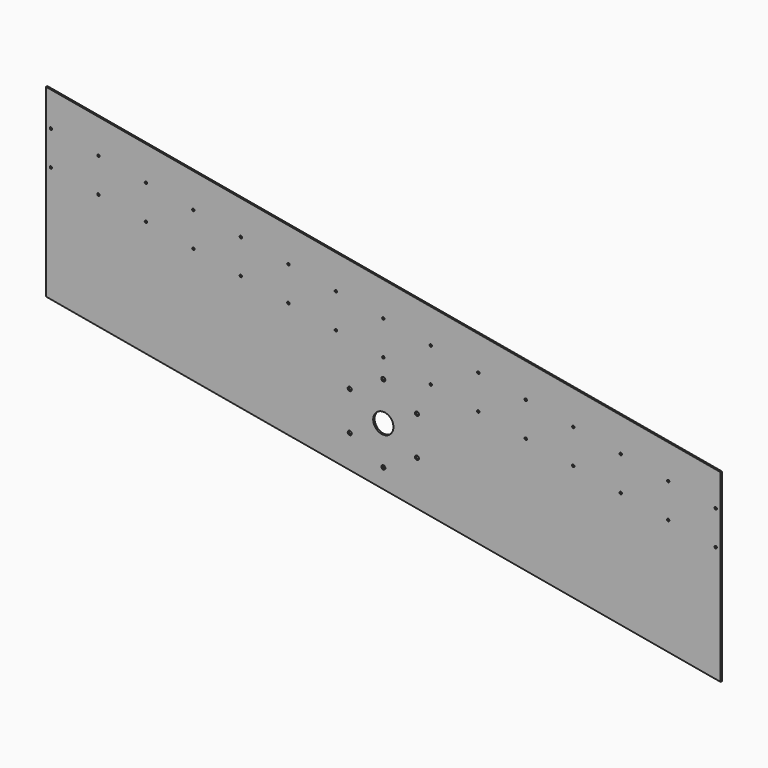
from build123d import *

# Parameters (mm, degrees)
F0_R     = 6
F0_R_2   = 30
F0_R_3   = 3.5
F1_DEPTH = 2.5


# Not quite as in the source:
# - a feature names something its author has since deleted; it is built from what else it names


with BuildPart() as f1:
    # F0 (on Front) → F1 (new body, symmetric)
    with BuildSketch(Plane.XZ):
        Polygon((0, 255), (1435, 0), (1435, 547.5993031359), (-565, 903), (-565, 355.4006968641), align=None)
        with Locations((335.4070785648, 292.4334004787)):
            Circle(F0_R, mode=Mode.SUBTRACT)
        with Locations((335.4070785648, 407.4334004787)):
            Circle(F0_R, mode=Mode.SUBTRACT)
        with Locations((435, 234.9334004787)):
            Circle(F0_R, mode=Mode.SUBTRACT)
        with Locations((534.5929214352, 292.4334004787)):
            Circle(F0_R, mode=Mode.SUBTRACT)
        with Locations((435, 349.9334004787)):
            Circle(F0_R_2, mode=Mode.SUBTRACT)
        with Locations((534.5929214352, 407.4334004787)):
            Circle(F0_R, mode=Mode.SUBTRACT)
        with Locations((857.3829507159, 447.1088550113)):
            Circle(F0_R_3, mode=Mode.SUBTRACT)
        with Locations((998.1772676211, 422.08965584)):
            Circle(F0_R_3, mode=Mode.SUBTRACT)
        with Locations((1138.9715845264, 397.0704566686)):
            Circle(F0_R_3, mode=Mode.SUBTRACT)
        with Locations((1279.7659014317, 372.0512574973)):
            Circle(F0_R_3, mode=Mode.SUBTRACT)
        with Locations((1420.560218337, 347.032058326)):
            Circle(F0_R_3, mode=Mode.SUBTRACT)
        with Locations((1420.560218337, 448.5986578473)):
            Circle(F0_R_3, mode=Mode.SUBTRACT)
        with Locations((-409.7659014317, 672.2816475532)):
            Circle(F0_R_3, mode=Mode.SUBTRACT)
        with Locations((-268.9715845264, 647.2624483819)):
            Circle(F0_R_3, mode=Mode.SUBTRACT)
        with Locations((-128.1772676211, 622.2432492105)):
            Circle(F0_R_3, mode=Mode.SUBTRACT)
        with Locations((294.2056830947, 547.1856516966)):
            Circle(F0_R_3, mode=Mode.SUBTRACT)
        with Locations((12.6170492841, 597.2240500392)):
            Circle(F0_R_3, mode=Mode.SUBTRACT)
        with Locations((153.4113661894, 572.2048508679)):
            Circle(F0_R_3, mode=Mode.SUBTRACT)
        with Locations((153.4113661894, 673.7714503892)):
            Circle(F0_R_3, mode=Mode.SUBTRACT)
        with Locations((294.2056830947, 648.7522512179)):
            Circle(F0_R_3, mode=Mode.SUBTRACT)
        with Locations((-550.560218337, 697.3008467245)):
            Circle(F0_R_3, mode=Mode.SUBTRACT)
        with Locations((-409.7659014317, 773.8482470745)):
            Circle(F0_R_3, mode=Mode.SUBTRACT)
        with Locations((-128.1772676211, 723.8098487319)):
            Circle(F0_R_3, mode=Mode.SUBTRACT)
        with Locations((-268.9715845264, 748.8290479032)):
            Circle(F0_R_3, mode=Mode.SUBTRACT)
        with Locations((-550.560218337, 798.8674462459)):
            Circle(F0_R_3, mode=Mode.SUBTRACT)
        with Locations((12.6170492841, 698.7906495606)):
            Circle(F0_R_3, mode=Mode.SUBTRACT)
        with Locations((435, 464.9334004787)):
            Circle(F0_R, mode=Mode.SUBTRACT)
        with Locations((575.7943169053, 497.1472533539)):
            Circle(F0_R_3, mode=Mode.SUBTRACT)
        with Locations((435, 522.1664525253)):
            Circle(F0_R_3, mode=Mode.SUBTRACT)
        with Locations((716.5886338106, 472.1280541826)):
            Circle(F0_R_3, mode=Mode.SUBTRACT)
        with Locations((857.3829507159, 548.6754545326)):
            Circle(F0_R_3, mode=Mode.SUBTRACT)
        with Locations((575.7943169053, 598.7138528753)):
            Circle(F0_R_3, mode=Mode.SUBTRACT)
        with Locations((435, 623.7330520466)):
            Circle(F0_R_3, mode=Mode.SUBTRACT)
        with Locations((716.5886338106, 573.694653704)):
            Circle(F0_R_3, mode=Mode.SUBTRACT)
        with Locations((1138.9715845264, 498.63705619)):
            Circle(F0_R_3, mode=Mode.SUBTRACT)
        with Locations((998.1772676211, 523.6562553613)):
            Circle(F0_R_3, mode=Mode.SUBTRACT)
        with Locations((1279.7659014317, 473.6178570187)):
            Circle(F0_R_3, mode=Mode.SUBTRACT)
    extrude(amount=F1_DEPTH, both=True)


solid = f1.part
